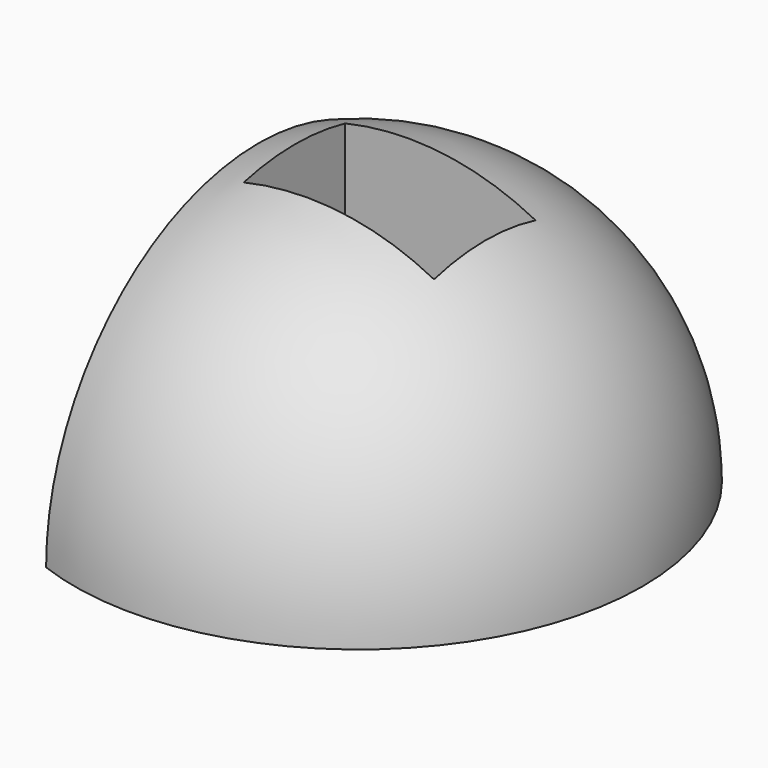
from build123d import *

# Parameters (mm, degrees)
F0_W          = 60
F0_H          = 40
F1_DEPTH      = 80
F4_W          = 60
F4_H          = 40
F5_DEPTH      = 25
F5_DEPTH_BACK = 80
F7_E7_W       = 192.0395717025
F7_E7_H       = 176.2685924768
F8_DEPTH      = 68.6223879457
F9_W          = 146.8224227428
F9_H          = 227.745719254
F10_DEPTH     = 104.3368522078


with BuildPart() as f1:
    # F0 (on Top) → F1 (new body)
    with BuildSketch(Plane.XY):
        with Locations((10, -0.2545155585)):
            Rectangle(F0_W, F0_H)
    extrude(amount=F1_DEPTH)

    # F2 (on Front) → F3 (revolve)
    with BuildSketch(Plane.XZ):
        with BuildLine():
            ThreePointArc((89.4427191, 0), (76.0845213036, 47.0228201834), (40, 80))
            Line((40, 80), (40, 0))
            Line((40, 0), (89.4427191, 0))
        make_face()
        with BuildLine():
            Line((40, 0), (40, 80))
            ThreePointArc((40, 80), (-47.0228201834, 76.0845213036), (-89.4427191, 0))
            Line((-89.4427191, 0), (40, 0))
        make_face()
    revolve(axis=Axis((0, 0, 0), (1, 0, 0)))

    # F4 (on face) → F5 (cut, two sides)
    with BuildSketch(Plane.XY.offset(80)) as f5_sk:
        with Locations((10, -0.2545155585)):
            Rectangle(F4_W, F4_H)
    extrude(amount=F5_DEPTH, mode=Mode.SUBTRACT)
    extrude(f5_sk.sketch, amount=-F5_DEPTH_BACK, mode=Mode.SUBTRACT)

    # F7_E7 (on explicit) → F8 (cut)
    with BuildSketch(Plane(origin=(-31.5267369151, 88.1342962384, 105.66496104), x_dir=(0, 0, -1), z_dir=(-1, 0, 0))):
        with Locations((96.0197858512, 88.1342962384)):
            Rectangle(F7_E7_W, F7_E7_H)
    extrude(amount=F8_DEPTH, mode=Mode.SUBTRACT)

    # F9 (on Top) → F10 (cut)
    with BuildSketch(Plane.XY):
        with Locations((26.485607028, 2.56710127)):
            Rectangle(F9_W, F9_H)
    extrude(amount=-F10_DEPTH, mode=Mode.SUBTRACT)


solid = f1.part
